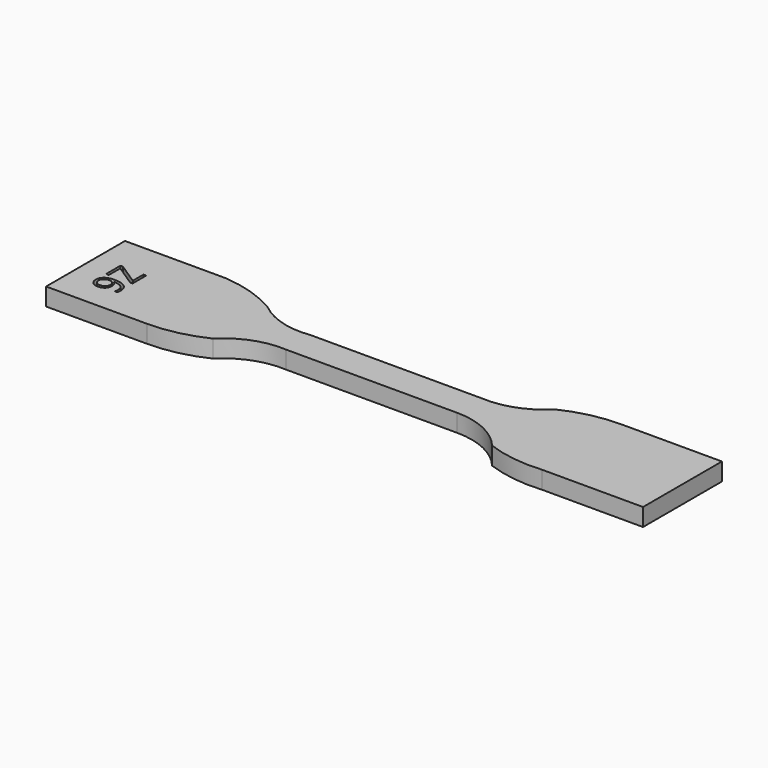
from build123d import *

# Parameters (mm, degrees)
F1_DEPTH     = 3.4
F2_TEXT_SIZE = 7.0564552314
F3_DEPTH     = 1


# Not quite as in the source:
# - Text() gives the source's letters only with a copy of the font that has no kerning and outlines rounded to 1/6400 em; it was checked with that copy


with BuildPart() as f1:
    # F0 (on Top) → F1 (new body)
    with BuildSketch(Plane.XY):
        with BuildLine():
            Line((-14.4320548165, 19.7811394548), (-33.8720548165, 19.7811394548))
            Line((-33.8720548165, 19.7811394548), (-33.8720548165, 0.7811394548))
            Line((-33.8720548165, 0.7811394548), (-14.4320548165, 0.7811394548))
            ThreePointArc((-14.4320548165, 0.7811394548), (-8.9053122052, 1.3996892086), (-3.6520548165, 3.2247301661))
            ThreePointArc((-3.6520548165, 3.2247301661), (1.3014698263, 6.4128780055), (7.1279451835, 7.2811394548))
            Line((7.1279451835, 7.2811394548), (40.1279451835, 7.2811394548))
            ThreePointArc((40.1279451835, 7.2811394548), (46.0837574042, 5.9511158081), (50.9079451835, 2.2137538538))
            ThreePointArc((50.9079451835, 2.2137538538), (56.2191047011, 0.9041953221), (61.6879451835, 0.7811394548))
            Line((61.6879451835, 0.7811394548), (81.1279451835, 0.7811394548))
            Line((81.1279451835, 0.7811394548), (81.1279451835, 19.7811394548))
            Line((81.1279451835, 19.7811394548), (61.6879451835, 19.7811394548))
            ThreePointArc((61.6879451835, 19.7811394548), (56.1612025723, 19.162589701), (50.9079451835, 17.3375487435))
            ThreePointArc((50.9079451835, 17.3375487435), (45.9544205407, 14.1494009041), (40.1279451835, 13.2811394548))
            Line((40.1279451835, 13.2811394548), (7.1279451835, 13.2811394548))
            ThreePointArc((7.1279451835, 13.2811394548), (1.4167452884, 13.6925537245), (-3.6520548165, 16.3560723447))
            ThreePointArc((-3.6520548165, 16.3560723447), (-8.8458057958, 18.686276846), (-14.4320548165, 19.7811394548))
        make_face()
    extrude(amount=F1_DEPTH)

    # F2 (on face) → F3 (cut)
    with BuildSketch(Plane.XY.offset(3.4)):
        with Locations(Location((-29.3720550835, 13.353464842), (0, 0, -90))):
            Text('Z6', F2_TEXT_SIZE, font='Open Sans', text_align=(TextAlign.LEFT, TextAlign.BOTTOM))
    extrude(amount=-F3_DEPTH, mode=Mode.SUBTRACT)


solid = f1.part
